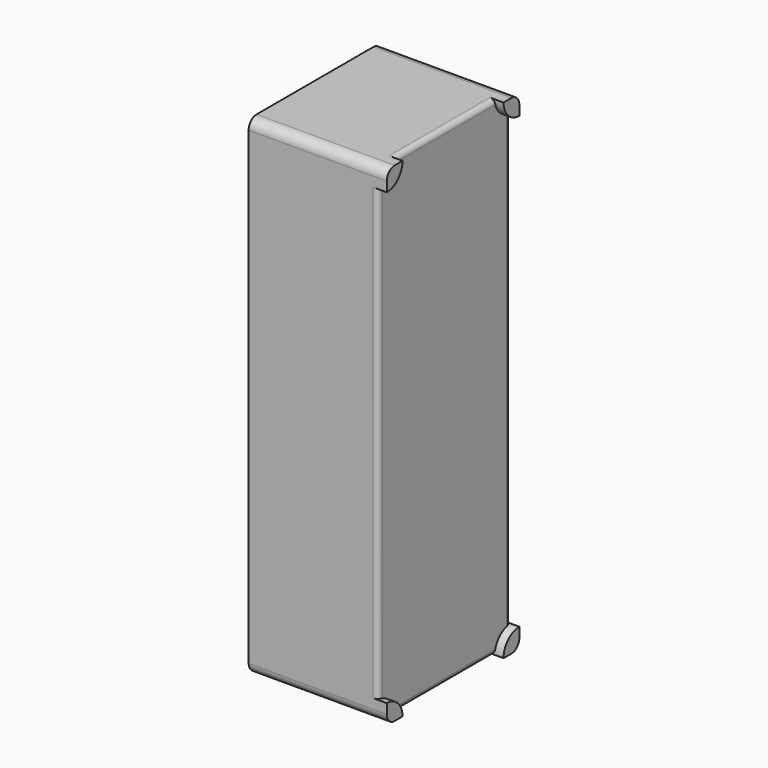
from build123d import *

# Parameters (mm, degrees)
F1_DEPTH = 1.524
F3_DEPTH = 40.132
F5_DEPTH = 2.794
F8_R     = 1.5875
F9_R     = 1.5875
F10_R    = 1.5875
F11_R    = 1.5875


with BuildPart() as f1:
    # F0 (on Right) → F1 (new body)
    with BuildSketch(Plane.YZ):
        with BuildLine():
            ThreePointArc((26.67, 75.565), (25.7400640303, 77.8100640303), (23.495, 78.74))
            Line((23.495, 78.74), (-23.495, 78.74))
            ThreePointArc((-23.495, 78.74), (-25.7400640303, 77.8100640303), (-26.67, 75.565))
            Line((-26.67, 75.565), (-26.67, -75.565))
            ThreePointArc((-26.67, -75.565), (-25.7400640303, -77.8100640303), (-23.495, -78.74))
            Line((-23.495, -78.74), (23.495, -78.74))
            ThreePointArc((23.495, -78.74), (25.7400640303, -77.8100640303), (26.67, -75.565))
            Line((26.67, -75.565), (26.67, 75.565))
        make_face()
    extrude(amount=F1_DEPTH)

    # F2 (on face) → F3 (join)
    with BuildSketch(Plane(origin=(0, 0, 0), x_dir=(0, -1, 0), z_dir=(-1, 0, 0))):
        with BuildLine():
            Line((23.495, 78.74), (-23.495, 78.74))
            ThreePointArc((-23.495, 78.74), (-25.7400640303, 77.8100640303), (-26.67, 75.565))
            Line((-26.67, 75.565), (-26.67, -75.565))
            ThreePointArc((-26.67, -75.565), (-25.7400640303, -77.8100640303), (-23.495, -78.74))
            Line((-23.495, -78.74), (23.495, -78.74))
            ThreePointArc((23.495, -78.74), (25.7400640303, -77.8100640303), (26.67, -75.565))
            Line((26.67, -75.565), (26.67, 75.565))
            ThreePointArc((26.67, 75.565), (25.7400640303, 77.8100640303), (23.495, 78.74))
        make_face()
        with BuildLine():
            ThreePointArc((25.146, -75.6285), (24.6810320151, -76.7510320151), (23.5585, -77.216))
            Line((23.5585, -77.216), (-23.5585, -77.216))
            ThreePointArc((-23.5585, -77.216), (-24.6810320151, -76.7510320151), (-25.146, -75.6285))
            Line((-25.146, -75.6285), (-25.146, 75.6285))
            ThreePointArc((-25.146, 75.6285), (-24.6810320151, 76.7510320151), (-23.5585, 77.216))
            Line((-23.5585, 77.216), (23.5585, 77.216))
            ThreePointArc((23.5585, 77.216), (24.6810320151, 76.7510320151), (25.146, 75.6285))
            Line((25.146, 75.6285), (25.146, -75.6285))
        make_face(mode=Mode.SUBTRACT)
    extrude(amount=F3_DEPTH)

    # F4 (on face) → F5 (join)
    with BuildSketch(Plane.YZ.offset(1.524)):
        with BuildLine():
            ThreePointArc((-26.67, 72.39), (-22.1798719395, 74.2498719395), (-20.32, 78.74))
            Line((-20.32, 78.74), (-23.495, 78.74))
            ThreePointArc((-23.495, 78.74), (-25.7400640303, 77.8100640303), (-26.67, 75.565))
            Line((-26.67, 75.565), (-26.67, 72.39))
        make_face()
    extrude(amount=F5_DEPTH)


with BuildPart() as f6_1:
    # F6: instance of F1
    add(f1.part.mirror(Plane.XY))


with BuildPart() as f1_1:
    add(f1.part)

    add(f6_1.part)  # F7 merges F6_1
    # F7: F6_1, F1 across plane
    add(f6_1.part.mirror(Plane.XZ))
    add(f1.part.mirror(Plane.XZ))

    # F8
    f8_edges = [f1_1.edges().sort_by_distance(p)[0] for p in [
        (1.524, -26.67, 0),
    ]]
    fillet(f8_edges, radius=F8_R)

    # F9
    f9_edges = [f1_1.edges().sort_by_distance(p)[0] for p in [
        (1.524, 0, -78.74),
    ]]
    fillet(f9_edges, radius=F9_R)

    # F10
    f10_edges = [f1_1.edges().sort_by_distance(p)[0] for p in [
        (1.524, 26.67, 0),
    ]]
    fillet(f10_edges, radius=F10_R)

    # F11
    f11_edges = [f1_1.edges().sort_by_distance(p)[0] for p in [
        (1.524, 0, 78.74),
    ]]
    fillet(f11_edges, radius=F11_R)


solid = f1_1.part
